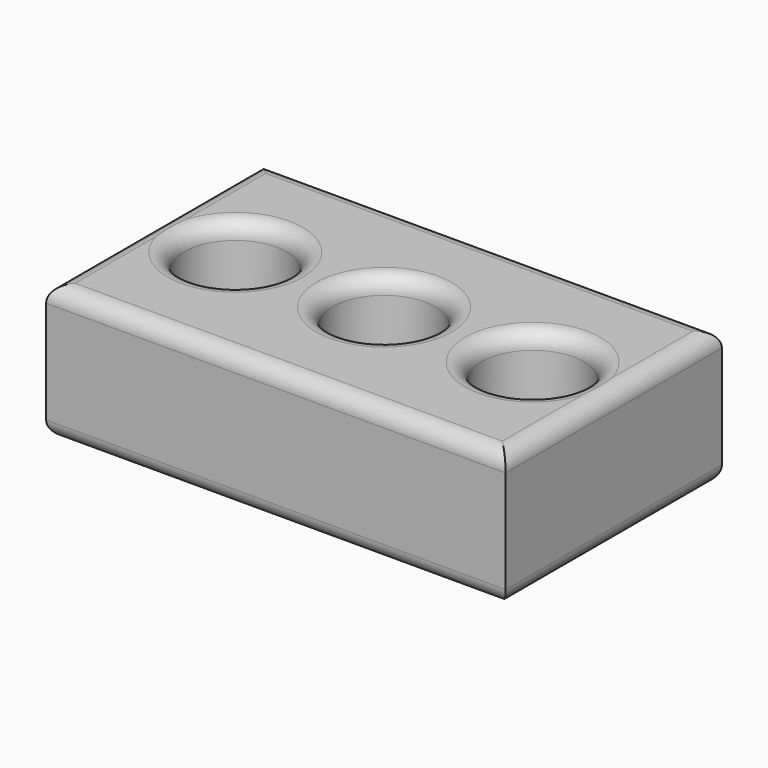
from build123d import *

# Parameters (mm, degrees)
F0_W        = 85
F0_H        = 50
F0_R        = 9.4896573641
F1_DEPTH    = 12.5
F2_T1_DEPTH = 100
F2_T3_DEPTH = 65


# Not quite as in the source:
# - a fillet or chamfer that OpenCascade refuses, or shapes differently, is made with other operations: its cross-section is extruded or revolved along the edge and cut away or added


with BuildPart() as f1:
    # F0 (on Top) → F1 (new body, symmetric)
    with BuildSketch(Plane.XY):
        Rectangle(F0_W, F0_H)
        with Locations((-27.5, 0)):
            Circle(F0_R, mode=Mode.SUBTRACT)
        Circle(F0_R, mode=Mode.SUBTRACT)
        with Locations((27.5, 0)):
            Circle(F0_R, mode=Mode.SUBTRACT)
    extrude(amount=F1_DEPTH, both=True)

    # F2: fillet of radius 3 on 14 edges, made by hand

    # F2_s2 → F2_t1 (cut)
    with BuildSketch(Plane.YZ.offset(-50)):
        with BuildLine():
            ThreePointArc((25, -9.5), (24.1213203436, -11.6213203436), (22, -12.5))
            Line((22, -12.5), (25, -12.5))
            Line((25, -12.5), (25, -9.5))
        make_face()
        with BuildLine():
            ThreePointArc((-25, -9.5), (-24.1213203436, -11.6213203436), (-22, -12.5))
            Line((-22, -12.5), (-25, -12.5))
            Line((-25, -12.5), (-25, -9.5))
        make_face()
        with BuildLine():
            ThreePointArc((25, 9.5), (24.1213203436, 11.6213203436), (22, 12.5))
            Line((22, 12.5), (25, 12.5))
            Line((25, 12.5), (25, 9.5))
        make_face()
        with BuildLine():
            ThreePointArc((-25, 9.5), (-24.1213203436, 11.6213203436), (-22, 12.5))
            Line((-22, 12.5), (-25, 12.5))
            Line((-25, 12.5), (-25, 9.5))
        make_face()
    extrude(amount=F2_T1_DEPTH, mode=Mode.SUBTRACT)

    # F2_s4 → F2_t3 (cut)
    with BuildSketch(Plane.XZ.offset(-32.5)):
        with BuildLine():
            ThreePointArc((-42.5, -9.5), (-41.6213203436, -11.6213203436), (-39.5, -12.5))
            Line((-39.5, -12.5), (-42.5, -12.5))
            Line((-42.5, -12.5), (-42.5, -9.5))
        make_face()
        with BuildLine():
            ThreePointArc((42.5, -9.5), (41.6213203436, -11.6213203436), (39.5, -12.5))
            Line((39.5, -12.5), (42.5, -12.5))
            Line((42.5, -12.5), (42.5, -9.5))
        make_face()
        with BuildLine():
            ThreePointArc((-39.5, 12.5), (-41.6213203436, 11.6213203436), (-42.5, 9.5))
            Line((-42.5, 9.5), (-42.5, 12.5))
            Line((-42.5, 12.5), (-39.5, 12.5))
        make_face()
        with BuildLine():
            ThreePointArc((42.5, 9.5), (41.6213203436, 11.6213203436), (39.5, 12.5))
            Line((39.5, 12.5), (42.5, 12.5))
            Line((42.5, 12.5), (42.5, 9.5))
        make_face()
    extrude(amount=F2_T3_DEPTH, mode=Mode.SUBTRACT)

    # F2_s5 → F2_t6 (revolve, cut)
    with BuildSketch(Plane.XZ):
        with BuildLine():
            ThreePointArc((36.9896573641, -9.5), (37.8683370205, -11.6213203436), (39.9896573641, -12.5))
            Line((39.9896573641, -12.5), (36.9896573641, -12.5))
            Line((36.9896573641, -12.5), (36.9896573641, -9.5))
        make_face()
    revolve(axis=Axis((27.5, 0, -12.5), (0, 0, 1)), mode=Mode.SUBTRACT)

    # F2_s7 → F2_t8 (revolve, cut)
    with BuildSketch(Plane.XZ):
        with BuildLine():
            ThreePointArc((9.4896573641, -9.5), (10.3683370205, -11.6213203436), (12.4896573641, -12.5))
            Line((12.4896573641, -12.5), (9.4896573641, -12.5))
            Line((9.4896573641, -12.5), (9.4896573641, -9.5))
        make_face()
    revolve(axis=Axis((0, 0, -12.5), (0, 0, 1)), mode=Mode.SUBTRACT)

    # F2_s9 → F2_t10 (revolve, cut)
    with BuildSketch(Plane.XZ):
        with BuildLine():
            ThreePointArc((-18.0103426359, -9.5), (-17.1316629795, -11.6213203436), (-15.0103426359, -12.5))
            Line((-15.0103426359, -12.5), (-18.0103426359, -12.5))
            Line((-18.0103426359, -12.5), (-18.0103426359, -9.5))
        make_face()
    revolve(axis=Axis((-27.5, 0, -12.5), (0, 0, 1)), mode=Mode.SUBTRACT)

    # F2_s11 → F2_t12 (revolve, cut)
    with BuildSketch(Plane.XZ):
        with BuildLine():
            ThreePointArc((39.9896573641, 12.5), (37.8683370205, 11.6213203436), (36.9896573641, 9.5))
            Line((36.9896573641, 9.5), (36.9896573641, 12.5))
            Line((36.9896573641, 12.5), (39.9896573641, 12.5))
        make_face()
    revolve(axis=Axis((27.5, 0, 12.5), (0, 0, 1)), mode=Mode.SUBTRACT)

    # F2_s13 → F2_t14 (revolve, cut)
    with BuildSketch(Plane.XZ):
        with BuildLine():
            ThreePointArc((12.4896573641, 12.5), (10.3683370205, 11.6213203436), (9.4896573641, 9.5))
            Line((9.4896573641, 9.5), (9.4896573641, 12.5))
            Line((9.4896573641, 12.5), (12.4896573641, 12.5))
        make_face()
    revolve(axis=Axis((0, 0, 12.5), (0, 0, 1)), mode=Mode.SUBTRACT)

    # F2_s15 → F2_t16 (revolve, cut)
    with BuildSketch(Plane.XZ):
        with BuildLine():
            ThreePointArc((-15.0103426359, 12.5), (-17.1316629795, 11.6213203436), (-18.0103426359, 9.5))
            Line((-18.0103426359, 9.5), (-18.0103426359, 12.5))
            Line((-18.0103426359, 12.5), (-15.0103426359, 12.5))
        make_face()
    revolve(axis=Axis((-27.5, 0, 12.5), (0, 0, 1)), mode=Mode.SUBTRACT)


solid = f1.part
